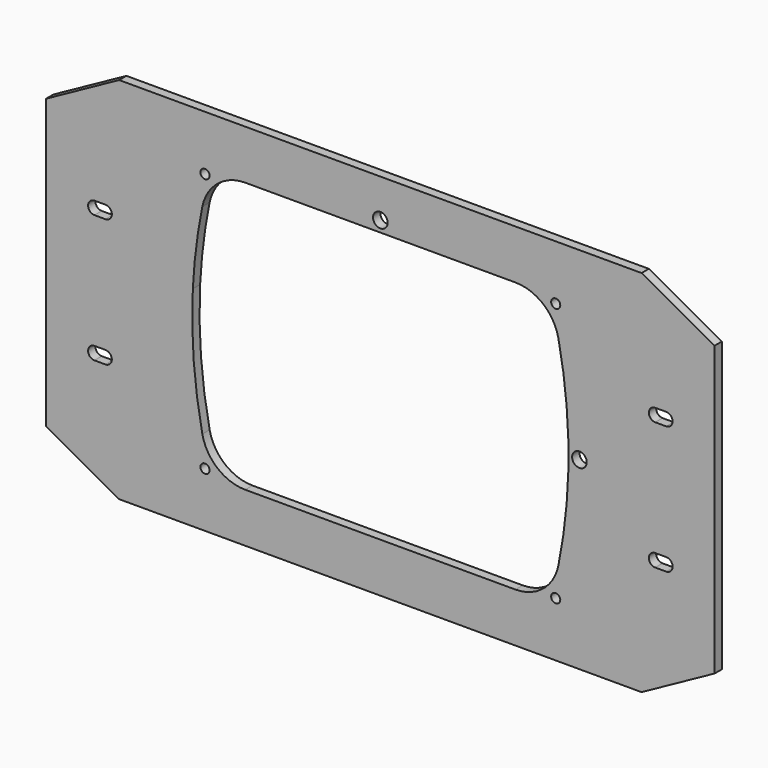
from build123d import *

# Parameters (mm, degrees)
F0_R     = 2.5
F0_R_2   = 4
F1_DEPTH = 5


with BuildPart() as f1:
    # F0 (on Front) → F1 (new body)
    with BuildSketch(Plane.XZ):
        Polygon((185.009293, 204.252433), (225.009293, 182.252433), (368.009293, 182.252433), (511.009293, 182.252433), (551.009293, 204.252433), (551.009293, 362.252433), (511.009293, 384.252433), (389.4801139832, 384.252433), (225.009293, 384.252433), (185.009293, 362.252433), align=None)
        with BuildLine():
            Line((211.509293, 251.752433), (217.509293, 251.752433))
            ThreePointArc((217.509293, 251.752433), (221.009293, 248.252433), (217.509293, 244.752433))
            Line((217.509293, 244.752433), (211.509293, 244.752433))
            ThreePointArc((211.509293, 244.752433), (208.009293, 248.252433), (211.509293, 251.752433))
        make_face(mode=Mode.SUBTRACT)
        with Locations((272.009293, 212.252433)):
            Circle(F0_R, mode=Mode.SUBTRACT)
        with BuildLine():
            ThreePointArc((270.5452164665, 338.0524329864), (278.8813852258, 351.8427530574), (294.060318, 357.252433))
            Line((294.060318, 357.252433), (388.009293, 357.252433))
            Line((388.009293, 357.252433), (441.958267, 357.252433))
            ThreePointArc((441.958267, 357.252433), (457.1371997667, 351.8427530635), (465.4733685296, 338.0524330052))
            ThreePointArc((465.4733685296, 338.0524330052), (469.9900217644, 306.8643277742), (470.8957123265, 275.3638866829))
            ThreePointArc((470.8957123265, 275.3638866829), (469.1970699877, 251.7911247549), (465.4733685296, 228.4524328857))
            ThreePointArc((465.4733685296, 228.4524328857), (457.1371997667, 214.6621128274), (441.958267, 209.2524328909))
            Line((441.958267, 209.2524328909), (368.0092925, 209.2524328909))
            Line((368.0092925, 209.2524328909), (294.060318, 209.2524328909))
            ThreePointArc((294.060318, 209.2524328909), (278.8813852287, 214.6621128311), (270.545216468, 228.4524328972))
            ThreePointArc((270.545216468, 228.4524328972), (265.7992173248, 262.4616912169), (265.3442938418, 296.797491833))
            ThreePointArc((265.3442938418, 296.797491833), (267.1610334487, 317.523764537), (270.5452164665, 338.0524329864))
        make_face(mode=Mode.SUBTRACT)
        with BuildLine():
            ThreePointArc((211.509293, 314.752433), (208.009293, 318.252433), (211.509293, 321.752433))
            Line((211.509293, 321.752433), (217.509293, 321.752433))
            ThreePointArc((217.509293, 321.752433), (221.009293, 318.252433), (217.509293, 314.752433))
            Line((217.509293, 314.752433), (211.509293, 314.752433))
        make_face(mode=Mode.SUBTRACT)
        with Locations((272.009293, 354.252433)):
            Circle(F0_R, mode=Mode.SUBTRACT)
        with Locations((368.009293, 363.252433)):
            Circle(F0_R_2, mode=Mode.SUBTRACT)
        with Locations((464.009293, 212.252433)):
            Circle(F0_R, mode=Mode.SUBTRACT)
        with BuildLine():
            Line((518.509293, 251.752433), (524.509293, 251.752433))
            ThreePointArc((524.509293, 251.752433), (528.009293, 248.252433), (524.509293, 244.752433))
            Line((524.509293, 244.752433), (518.509293, 244.752433))
            ThreePointArc((518.509293, 244.752433), (515.009293, 248.252433), (518.509293, 251.752433))
        make_face(mode=Mode.SUBTRACT)
        with Locations((477.009293, 283.252433)):
            Circle(F0_R_2, mode=Mode.SUBTRACT)
        with BuildLine():
            Line((524.509293, 314.752433), (518.509293, 314.752433))
            ThreePointArc((518.509293, 314.752433), (515.009293, 318.252433), (518.509293, 321.752433))
            Line((518.509293, 321.752433), (524.509293, 321.752433))
            ThreePointArc((524.509293, 321.752433), (528.009293, 318.252433), (524.509293, 314.752433))
        make_face(mode=Mode.SUBTRACT)
        with Locations((464.009293, 354.252433)):
            Circle(F0_R, mode=Mode.SUBTRACT)
    extrude(amount=F1_DEPTH)


solid = f1.part
